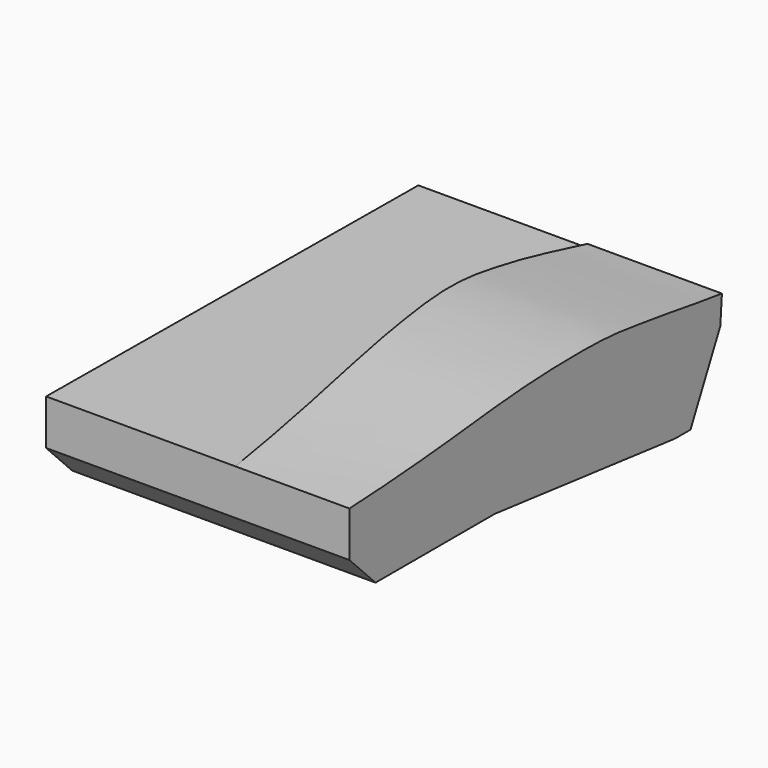
from build123d import *

# Parameters (mm, degrees)
F1_DEPTH      = 41.35
F3_DEPTH      = 25
F5_END_RADIUS = 74.802
F5_REACH      = 106.3335182113


# Not quite as in the source:
# - the dataset's text gives a spline's control points without its knots; the knots are read off the source's solid


with BuildPart() as f1:
    # F0 (on Right) → F1 (new body)
    with BuildSketch(Plane.YZ):
        with BuildLine():
            Line((63.1800009416, -8.0976060032), (63.4529719416, -4.2942040032))
            add(Edge.make_bspline(
                [(63.4529719416, -4.2942040032), (60.5909509416, -3.9429730032), (55.6489039416, -3.1055340032), (49.4296259416, -2.2738210032), (43.3081119416, -1.3786650032), (29.5308939416, -1.6169810032), (17.1469639416, -3.1247220032), (6.4803219416, -3.9842320032), (0.4299239416, -4.2745560032), (-5.84e-08, -4.2942040032)],
                knots=[26.768967, 26.768967, 26.768967, 26.768967, 180.626612, 384.452895, 590.22148, 806.300894, 1087.362377, 1488.926341, 1519.790594, 1519.790594, 1519.790594, 1519.790594], degree=3))
            Line((-5.84e-08, -4.2942040032), (-5.84e-08, -10.4802040032))
            Line((-5.84e-08, -10.4802040032), (4.4423189416, -15.0000000032))
            Line((4.4423189416, -15.0000000032), (24.7692139896, -15.0000000178))
            Line((24.7692139896, -15.0000000178), (55.4551508606, -18.4565160095))
            Line((55.4551508606, -18.4565160095), (58.0976629416, -18.4565160032))
            Line((58.0976629416, -18.4565160032), (63.1800009416, -8.0976060032))
        make_face()
    extrude(amount=F1_DEPTH)

    # F2 (on Top) → F3 (cut)
    with BuildSketch(Plane.XY):
        with BuildLine():
            Line((0, -5.84e-08), (25.795, -5.84e-08))
            Line((25.795, -5.84e-08), (21.4260625948, 37.7077443179))
            ThreePointArc((21.4260625948, 37.7077443179), (21.1044219976, 50.6495390339), (23.019, 63.4529719416))
            Line((23.019, 63.4529719416), (0, 63.4529719416))
            Line((0, 63.4529719416), (0, -5.84e-08))
        make_face()
    extrude(amount=-F3_DEPTH, mode=Mode.SUBTRACT)

    f5_end = (Plane(origin=(95.763650211, 46.0301400912, -9.9833453774), x_dir=(1, 0, 0), z_dir=(0, 0, 1)) * Cylinder(F5_END_RADIUS, 350.2040983296, mode=Mode.PRIVATE)).faces().sort_by_distance((21.1044219976, 50.6495390339, -9.9833453774))[0]
    # F4 (on Right) → F5 (join, up to the whole of a round face its end follows)
    with BuildSketch(Plane.YZ):
        Polygon((63.1800009416, -8.0976060032), (63.4204743857, -4.7470040032), (-5.84e-08, -4.2942040032), (-5.84e-08, -10.4802040032), (4.4423189416, -15.0000000032), (24.7692139896, -15.0000000178), (37.7077443179, -16.4574180258), (55.4551508606, -18.4565160095), (58.0976629416, -18.4565160032), align=None)
    f5_long = extrude(amount=F5_REACH, mode=Mode.PRIVATE)
    add(split(f5_long, bisect_by=f5_end, keep=Keep.TOP, mode=Mode.PRIVATE))


solid = f1.part
